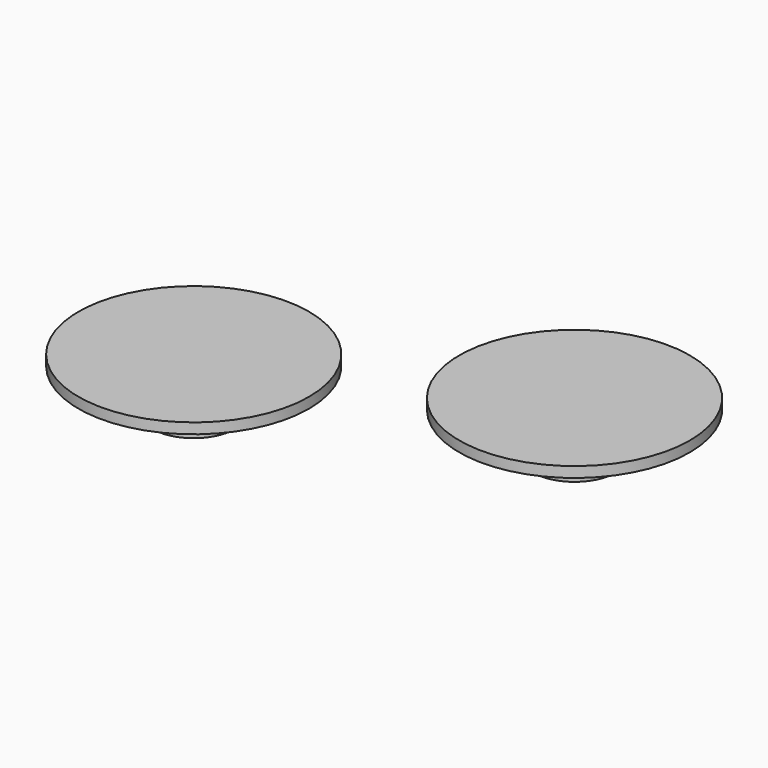
from build123d import *

# Parameters (mm, degrees)
F0_R     = 11
F0_R_2   = 6
F0_R_3   = 3.95
F1_DEPTH = 1
F2_DEPTH = 4
F3_DEPTH = 1


with BuildPart() as f1:
    # F0 (on Top) → F1 (new body)
    with BuildSketch(Plane.XY):
        with Locations((-32.5816608965, 7.518844679)):
            Circle(F0_R)
        with Locations((-32.5816608965, 7.518844679)):
            Circle(F0_R_2, mode=Mode.SUBTRACT)
        with Locations((-32.5816608965, 7.518844679)):
            Circle(F0_R_2)
        with Locations((-32.5816608965, 7.518844679)):
            Circle(F0_R_3, mode=Mode.SUBTRACT)
        with Locations((-32.5816608965, 7.518844679)):
            Circle(F0_R_3)
    extrude(amount=F1_DEPTH)

    # F0 (on Top) → F2 (join)
    with BuildSketch(Plane.XY):
        with Locations((-32.5816608965, 7.518844679)):
            Circle(F0_R_3)
    extrude(amount=-F2_DEPTH)

    # F0 (on Top) → F3 (join)
    with BuildSketch(Plane.XY):
        with Locations((-32.5816608965, 7.518844679)):
            Circle(F0_R_2)
        with Locations((-32.5816608965, 7.518844679)):
            Circle(F0_R_3, mode=Mode.SUBTRACT)
    extrude(amount=-F3_DEPTH)


with BuildPart() as f1b:
    # F0 (on Top) → F1, piece 2 (new body)
    with BuildSketch(Plane.XY):
        with Locations((-6.0249380767, 19.7376422584)):
            Circle(F0_R)
        with Locations((-6.0249380767, 19.7376422584)):
            Circle(F0_R_2, mode=Mode.SUBTRACT)
        with Locations((-6.0249380767, 19.7376422584)):
            Circle(F0_R_2)
        with Locations((-6.0249380767, 19.7376422584)):
            Circle(F0_R_3, mode=Mode.SUBTRACT)
        with Locations((-6.0249380767, 19.7376422584)):
            Circle(F0_R_3)
    extrude(amount=F1_DEPTH)


with BuildPart() as f2:
    # F0 (on Top) → F2, piece 2 (new body)
    with BuildSketch(Plane.XY):
        with Locations((-6.0249380767, 19.7376422584)):
            Circle(F0_R_3)
    extrude(amount=-F2_DEPTH)


with BuildPart() as f3:
    # F0 (on Top) → F3, piece 2 (new body)
    with BuildSketch(Plane.XY):
        with Locations((-6.0249380767, 19.7376422584)):
            Circle(F0_R_2)
        with Locations((-6.0249380767, 19.7376422584)):
            Circle(F0_R_3, mode=Mode.SUBTRACT)
    extrude(amount=-F3_DEPTH)


solid = Compound([f1.part, f1b.part, f2.part, f3.part])
